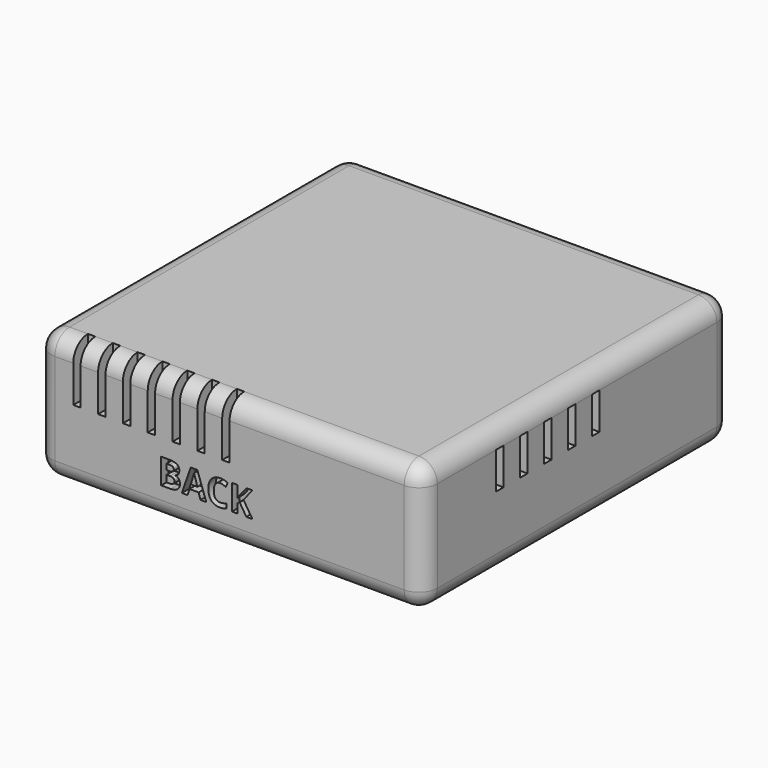
from build123d import *

# Parameters (mm, degrees)
F0_W         = 210
F0_H         = 210
F1_DEPTH     = 70
F2_R         = 10
F3_R         = 10
F4_W         = 4
F4_H         = 30
F5_DEPTH     = 10
F6_W         = 5
F6_H         = 20
F7_DEPTH     = 5
F8_TEXT_SIZE = 19.2795802529
F9_DEPTH     = 5


# Not quite as in the source:
# - Text() gives the source's letters only with a copy of the font that has no kerning and outlines rounded to 1/6400 em; it was checked with that copy


with BuildPart() as f1:
    # F0 (on Top) → F1 (new body)
    with BuildSketch(Plane.XY):
        Rectangle(F0_W, F0_H)
    extrude(amount=F1_DEPTH)

    # F2
    f2_edges = [f1.edges().sort_by_distance(p)[0] for p in [
        (-105, 105, 35),
        (105, 105, 35),
        (-105, -105, 35),
        (105, -105, 35),
    ]]
    fillet(f2_edges, radius=F2_R)

    # F3
    f3_edges = [f1.edges().sort_by_distance(p)[0] for p in [
        (105, 0, 70),
        (105, 0, 0),
    ]]
    fillet(f3_edges, radius=F3_R)

    # F4 (on face) → F5 (cut)
    with BuildSketch(Plane.XZ.offset(105)):
        with Locations((-83, 55)):
            Rectangle(F4_W, F4_H)
        with Locations((-2, 55)):
            Rectangle(F4_W, F4_H)
        with Locations((-69.5, 55)):
            Rectangle(F4_W, F4_H)
        with Locations((-56, 55)):
            Rectangle(F4_W, F4_H)
        with Locations((-42.5, 55)):
            Rectangle(F4_W, F4_H)
        with Locations((-29, 55)):
            Rectangle(F4_W, F4_H)
        with Locations((-15.5, 55)):
            Rectangle(F4_W, F4_H)
    extrude(amount=-F5_DEPTH, mode=Mode.SUBTRACT)

    # F6 (on face) → F7 (cut)
    with BuildSketch(Plane.YZ.offset(105)):
        with Locations((-52.5, 50)):
            Rectangle(F6_W, F6_H)
        with Locations((-36.2, 50)):
            Rectangle(F6_W, F6_H)
        with Locations((-19.9, 50)):
            Rectangle(F6_W, F6_H)
        with Locations((-3.6, 50)):
            Rectangle(F6_W, F6_H)
        with Locations((12.7, 50)):
            Rectangle(F6_W, F6_H)
    extrude(amount=-F7_DEPTH, mode=Mode.SUBTRACT)

    # F8 (on face) → F9 (cut)
    with BuildSketch(Plane.XZ.offset(105)):
        with Locations((-38.9220751822, 17.0359667391)):
            Text('BACK', F8_TEXT_SIZE, font='Open Sans', font_style=FontStyle.BOLD, text_align=(TextAlign.LEFT, TextAlign.BOTTOM))
    extrude(amount=-F9_DEPTH, mode=Mode.SUBTRACT)


solid = f1.part
